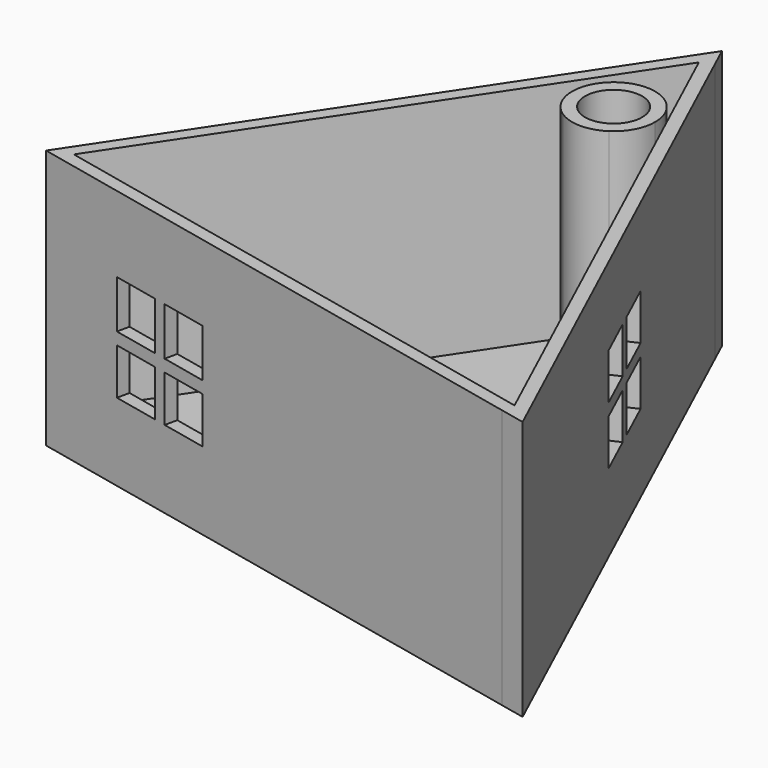
from build123d import *

# Parameters (mm, degrees)
F1_DEPTH = 38.1
F0_R     = 4.191
F2_DEPTH = 5.08
F3_W     = 6.9084239401
F3_H     = 7.0400872709
F3_H_2   = 6.7767606093
F4_DEPTH = 1.905
F5_W     = 6.731
F5_H     = 6.731
F6_DEPTH = 2.54


# Not quite as in the source:
# - a feature names something its author has since deleted; it is built from what else it names


with BuildPart() as f1:
    # F0 (on Top) → F1 (new body)
    with BuildSketch(Plane.XY):
        Polygon((0.3095794826, 51.1243626163), (-43.2167308403, -14.2446323873), (-44.7347259133, -16.5243986163), (36.2745233354, -34.199096887), (39.9642340225, -35.0041225317), (1.7162043522, 48.0692239296), align=None)
        Polygon((-41.6572931301, -15.282992694), (0, 47.2790615276), (36.6729057896, -32.3731724479), align=None, mode=Mode.SUBTRACT)
    extrude(amount=F1_DEPTH)

    # F3 (on face) → F4 (cut)
    with BuildSketch(Plane(origin=(-5.4742330467, -25.0903015448, 0), x_dir=(0.9770158795, -0.2131665339, 0), z_dir=(-0.2131665339, -0.9770158795, 0))):
        with Locations((-23.8466220251, 23.4590436355)):
            Rectangle(F3_W, F3_H)
        with Locations((-23.8466220251, 14.7726196953)):
            Rectangle(F3_W, F3_H_2)
        with Locations((-15.1601980849, 14.7726196953)):
            Rectangle(F3_W, F3_H_2)
        with Locations((-15.1601980849, 23.4590436355)):
            Rectangle(F3_W, F3_H)
    extrude(amount=-F4_DEPTH, mode=Mode.SUBTRACT)

    # F5 (on face) → F6 (cut)
    with BuildSketch(Plane(origin=(19.6768020366, 9.0594509571, 0), x_dir=(-0.4182150426, 0.908348049, 0), z_dir=(0.908348049, 0.4182150426, 0))):
        with Locations((-4.2545, 23.3045)):
            Rectangle(F5_W, F5_H)
        with Locations((-4.2545, 14.7955)):
            Rectangle(F5_W, F5_H)
        with Locations((4.2545, 14.7955)):
            Rectangle(F5_W, F5_H)
        with Locations((4.2545, 23.3045)):
            Rectangle(F5_W, F5_H)
    extrude(amount=-F6_DEPTH, mode=Mode.SUBTRACT)


with BuildPart() as f1b:
    # F0 (on Top) → F1, piece 2 (new body)
    with BuildSketch(Plane.XY):
        with BuildLine():
            ThreePointArc((2.6368516072, 27.5348942884), (4.6181244636, 29.726524701), (5.3347704338, 32.5927250691))
            ThreePointArc((5.3347704338, 32.5927250691), (-3.6213867329, 37.9660358976), (-4.1472243368, 27.5348942884))
            ThreePointArc((-4.1472243368, 27.5348942884), (-0.7551863648, 26.5027682705), (2.6368516072, 27.5348942884))
        make_face()
        with Locations((-0.7551863648, 32.5927250691)):
            Circle(F0_R, mode=Mode.SUBTRACT)
    extrude(amount=F1_DEPTH)


with BuildPart() as f2:
    # F0 (on Top) → F2 (new body)
    with BuildSketch(Plane.XY):
        Polygon((36.6729057896, -32.3731724479), (0, 47.2790615276), (-41.6572931301, -15.282992694), align=None)
        with BuildLine():
            ThreePointArc((-4.1472243368, 27.5348942884), (-3.6213867329, 37.9660358976), (5.3347704338, 32.5927250691))
            ThreePointArc((5.3347704338, 32.5927250691), (4.6181244636, 29.726524701), (2.6368516072, 27.5348942884))
            Line((2.6368516072, 27.5348942884), (2.6368516072, 21.4253379491))
            Line((2.6368516072, 21.4253379491), (-0.7551863648, 21.4253379491))
            Line((-0.7551863648, 21.4253379491), (-4.1472243368, 21.4253379491))
            Line((-4.1472243368, 21.4253379491), (-4.1472243368, 27.5348942884))
        make_face(mode=Mode.SUBTRACT)
    extrude(amount=F2_DEPTH)


solid = Compound([f1.part, f1b.part, f2.part])
